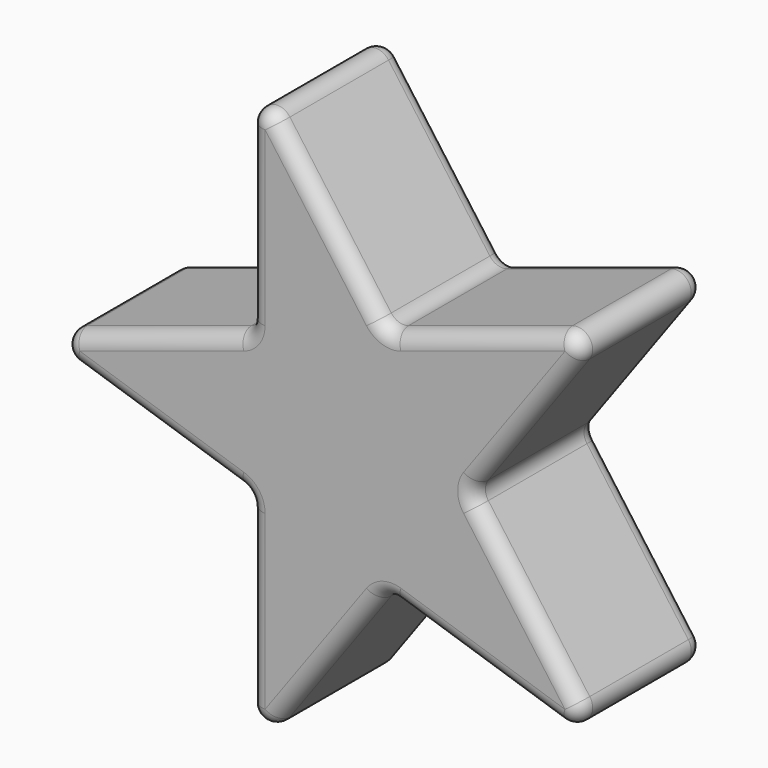
from build123d import *

# Parameters (mm, degrees)
F1_DEPTH = 50.8
F2_F1_R  = 5.08
F2_F2_R  = 5.08


with BuildPart() as f1:
    # F0 (on Front) → F1 (new body)
    with BuildSketch(Plane.XZ):
        Polygon((44.7892362247, -61.6470949714), (0, 0), (44.7892362247, 61.6470949714), (-27.681270317, 38.1), (-72.4705065417, 99.7470949714), (-72.4705065417, 23.5470949714), (-144.9410130834, 0), (-72.4705065417, -23.5470949714), (-72.4705065417, -99.7470949714), (-27.681270317, -38.1), align=None)
    extrude(amount=-F1_DEPTH)

    # F2: fillet of radius 5.08 on 21 edges, made by hand

    # F2_f1
    f2_f1_edges = [f1.edges().sort_by_distance(p)[0] for p in [
        (-27.681270317, 25.4, -38.1),
        (-72.4705065417, 25.4, -23.5470949714),
        (-72.4705065417, 25.4, 23.5470949714),
        (-27.681270317, 25.4, 38.1),
        (0, 25.4, 0),
    ]]
    fillet(f2_f1_edges, radius=F2_F1_R)

    # F2_f2
    f2_f2_edges = [f1.edges().sort_by_distance(p)[0] for p in [
        (-72.4705065417, 25.4, 99.7470949714),
        (-144.9410130834, 25.4, 0),
        (44.7892362247, 25.4, 61.6470949714),
        (44.7892362247, 25.4, -61.6470949714),
        (-72.4705065417, 25.4, -99.7470949714),
        (-72.4705065417, 50.8, -63.4925129925),
        (-51.1605979265, 50.8, -70.4165220265),
        (10.3090797881, 50.8, -50.4438130159),
        (-110.4608566468, 50.8, 11.2032819554),
        (-51.1605979265, 50.8, 70.4165220265),
        (23.4793276095, 50.8, 32.3165220265),
        (23.4793276095, 0, 32.3165220265),
        (10.3090797881, 0, 50.4438130159),
        (-72.4705065417, 0, 63.4925129925),
        (-110.4608566468, 0, -11.2032819554),
        (-51.1605979265, 0, -70.4165220265),
        (-27.3106893113, 0, -39.2405310605),
        (-73.4407002103, 0, -24.251981932),
        (-73.4407002103, 0, 24.251981932),
        (-27.3106893113, 0, 39.2405310605),
        (1.1992253257, 0, 0),
        (1.1992253257, 50.8, 0),
        (-27.3106893113, 50.8, 39.2405310605),
        (-73.4407002103, 50.8, 24.251981932),
        (-27.3106893113, 50.8, -39.2405310605),
        (-73.4407002103, 50.8, -24.251981932),
    ]]
    fillet(f2_f2_edges, radius=F2_F2_R)


solid = f1.part
